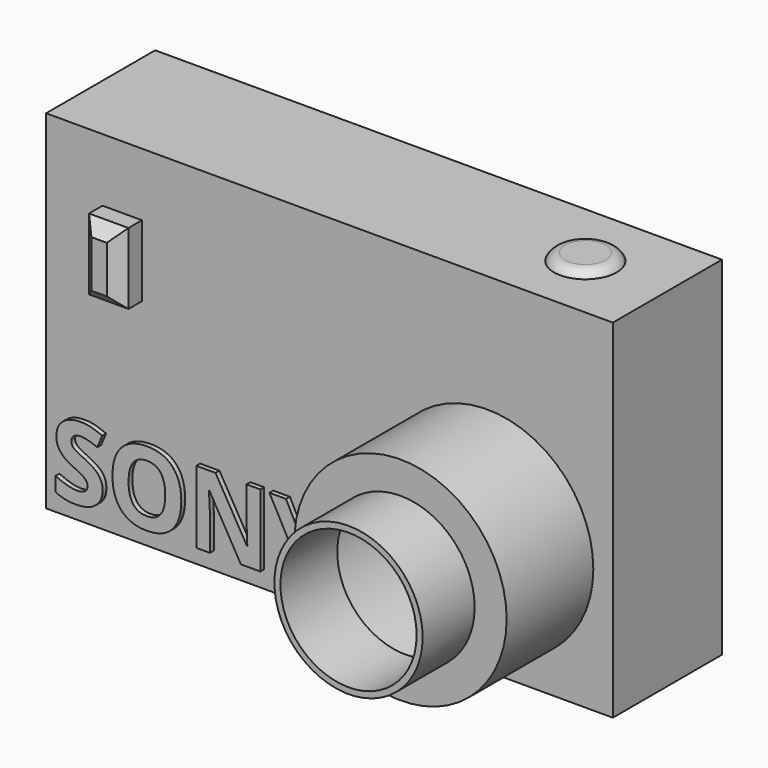
from build123d import *

# Parameters (mm, degrees)
F0_W          = 235.4213818908
F0_H          = 144.4907560945
F1_DEPTH      = 56.642
F2_R          = 44.082540145
F3_DEPTH      = 45
F4_R          = 30.7915579993
F5_DEPTH      = 27
F6_T          = -2.5
F7_R          = 13.018436694
F8_DEPTH      = 3
F10_W         = 16.3686871529
F10_H         = 29.5980665833
F11_DEPTH     = 12
F12_SIZE      = 5
F13_TEXT_SIZE = 42.0433831298
F14_DEPTH     = 2


# Not quite as in the source:
# - a fillet or chamfer that OpenCascade refuses, or shapes differently, is made with other operations: its cross-section is extruded or revolved along the edge and cut away or added
# - Text() gives the source's letters only with a copy of the font that has no kerning and outlines rounded to 1/6400 em; it was checked with that copy


with BuildPart() as f1:
    # F0 (on Front) → F1 (new body)
    with BuildSketch(Plane.XZ):
        with Locations((0.83482638, -1.5105344355)):
            Rectangle(F0_W, F0_H)
    extrude(amount=F1_DEPTH)

    # F2 (on face) → F3 (join)
    with BuildSketch(Plane.XZ.offset(56.642)):
        with Locations((66.3591846824, -22.0442321151)):
            Circle(F2_R)
    extrude(amount=F3_DEPTH)

    # F4 (on face) → F5 (join)
    with BuildSketch(Plane.XZ.offset(101.642)):
        with Locations((66.3591846824, -22.0442321151)):
            Circle(F4_R)
    extrude(amount=F5_DEPTH)

    # F6
    f6_openings = [f1.faces().sort_by_distance(p)[0] for p in [
        (66.359185, -128.642, -22.044232),
    ]]
    offset(amount=F6_T, openings=f6_openings, kind=Kind.INTERSECTION)

    # F7 (on face) → F8 (join)
    with BuildSketch(Plane.XY.offset(70.7348436117)):
        with Locations((84.4641178846, -28.321)):
            Circle(F7_R)
    extrude(amount=F8_DEPTH)

    # F9: fillet of radius 5 on 1 edges, made by hand

    # F9_s1 → F9_t2 (revolve, cut)
    with BuildSketch(Plane.XZ.offset(28.321)):
        with BuildLine():
            ThreePointArc((97.4825545787, 70.7348436117), (95.6385916712, 72.9181437444), (92.8999788837, 73.7348436117))
            Line((92.8999788837, 73.7348436117), (97.4825545787, 73.7348436117))
            Line((97.4825545787, 73.7348436117), (97.4825545787, 70.7348436117))
        make_face()
    revolve(axis=Axis((84.4641178846, -28.321, 73.7348436117), (0, 0, 1)), mode=Mode.SUBTRACT)

    # F10 (on face) → F11 (join)
    with BuildSketch(Plane.XZ.offset(56.642)):
        with Locations((-85.2493494749, 29.7567462549)):
            Rectangle(F10_W, F10_H)
    extrude(amount=F11_DEPTH)

    # F12
    f12_edges = [f1.edges().sort_by_distance(p)[0] for p in [
        (-85.249349, -68.642, 44.55578),
        (-93.433693, -68.642, 29.756746),
        (-85.249349, -68.642, 14.957713),
        (-77.065006, -68.642, 29.756746),
    ]]
    chamfer(f12_edges, length=F12_SIZE)

    # F13 (on face) → F14 (join)
    with BuildSketch(Plane.XZ.offset(56.642)):
        with Locations((-113.2949674502, -66.5746182203)):
            Text('SONY', F13_TEXT_SIZE, font='Open Sans', font_style=FontStyle.BOLD, text_align=(TextAlign.LEFT, TextAlign.BOTTOM))
    extrude(amount=F14_DEPTH)


solid = f1.part
